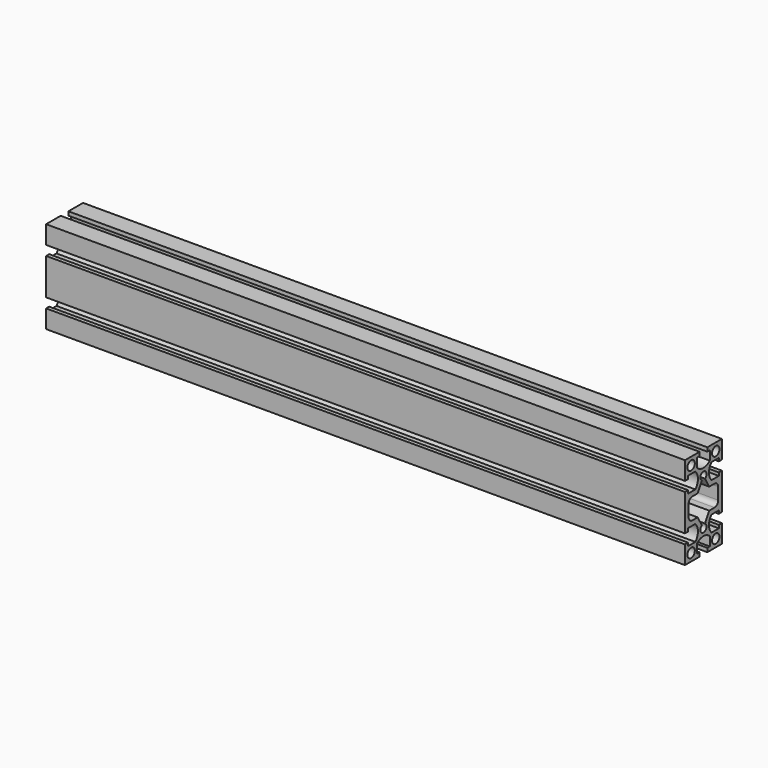
from build123d import *

# Parameters (mm, degrees)
F0_R     = 3
F1_DEPTH = 415


# Not quite as in the source:
# - ends of sketch curves that miss each other by under 0.0002 mm in the source are joined


with BuildPart() as f1:
    # F0 (on Right) → F1 (new body)
    with BuildSketch(Plane.YZ):
        with BuildLine():
            Line((12.5, -11.85), (15, -11.85))
            Line((15, -11.85), (15, 11.85))
            Line((15, 11.85), (12.5, 11.85))
            Line((12.5, 11.85), (12.5, 9.85))
            Line((12.5, 9.85), (6.547707, 9.85))
            ThreePointArc((6.5477069495, 9.8499999523), (4.5, 15), (6.5477069495, 20.1500000477))
            Line((6.547707, 20.15), (12.5, 20.15))
            Line((12.5, 20.15), (12.5, 18.15))
            Line((12.5, 18.15), (15, 18.15))
            Line((15, 18.15), (15, 30))
            Line((15, 30), (3.15, 30))
            Line((3.15, 30), (3.15, 27.5))
            Line((3.15, 27.5), (5.15, 27.5))
            Line((5.15, 27.5), (5.15, 21.547707))
            ThreePointArc((5.1500000477, 21.5477069495), (0, 19.5), (-5.1500000477, 21.5477069495))
            Line((-5.15, 21.547707), (-5.15, 27.5))
            Line((-5.15, 27.5), (-3.15, 27.5))
            Line((-3.15, 27.5), (-3.15, 30))
            Line((-3.15, 30), (-15, 30))
            Line((-15, 30), (-15, 18.15))
            Line((-15, 18.15), (-12.5, 18.15))
            Line((-12.5, 18.15), (-12.5, 20.15))
            Line((-12.5, 20.15), (-6.547707, 20.15))
            ThreePointArc((-6.5477069495, 20.1500000477), (-4.5, 15), (-6.5477069495, 9.8499999523))
            Line((-6.547707, 9.85), (-12.5, 9.85))
            Line((-12.5, 9.85), (-12.5, 11.85))
            Line((-12.5, 11.85), (-15, 11.85))
            Line((-15, 11.85), (-15, -11.85))
            Line((-15, -11.85), (-12.5, -11.85))
            Line((-12.5, -11.85), (-12.5, -9.85))
            Line((-12.5, -9.85), (-6.547707, -9.85))
            ThreePointArc((-6.5477069495, -9.8499999523), (-4.5, -15), (-6.5477069495, -20.1500000477))
            Line((-6.547707, -20.15), (-12.5, -20.15))
            Line((-12.5, -20.15), (-12.5, -18.15))
            Line((-12.5, -18.15), (-15, -18.15))
            Line((-15, -18.15), (-15, -30))
            Line((-15, -30), (-3.15, -30))
            Line((-3.15, -30), (-3.15, -27.5))
            Line((-3.15, -27.5), (-5.15, -27.5))
            Line((-5.15, -27.5), (-5.15, -21.547707))
            ThreePointArc((-5.1500000477, -21.5477069495), (0, -19.5), (5.1500000477, -21.5477069495))
            Line((5.15, -21.547707), (5.15, -27.5))
            Line((5.15, -27.5), (3.15, -27.5))
            Line((3.15, -27.5), (3.15, -30))
            Line((3.15, -30), (15, -30))
            Line((15, -30), (15, -18.15))
            Line((15, -18.15), (12.5, -18.15))
            Line((12.5, -18.15), (12.5, -20.15))
            Line((12.5, -20.15), (6.547707, -20.15))
            ThreePointArc((6.5477069495, -20.1500000477), (4.5, -15), (6.5477069495, -9.8499999523))
            Line((6.547707, -9.85), (12.5, -9.85))
            Line((12.5, -9.85), (12.5, -11.85))
        make_face()
        with Locations((-10, -25)):
            Circle(F0_R, mode=Mode.SUBTRACT)
        with Locations((10, -25)):
            Circle(F0_R, mode=Mode.SUBTRACT)
        with Locations((-10, 25)):
            Circle(F0_R, mode=Mode.SUBTRACT)
        with BuildLine():
            ThreePointArc((-12, 3.85), (-11.1213203436, 5.9713203436), (-9, 6.85))
            Line((-9, 6.85), (-4.705405, 6.85))
            Line((-4.705405, 6.85), (-1.25, 12.834936))
            ThreePointArc((-1.25, 12.834936), (0, 17.5), (1.2499997876, 12.8349363679))
            Line((1.2499997876, 12.8349363679), (4.705405, 6.85))
            Line((4.705405, 6.85), (9, 6.85))
            ThreePointArc((9, 6.85), (11.1213203436, 5.9713203436), (12, 3.85))
            Line((12, 3.85), (12, -3.85))
            ThreePointArc((12, -3.85), (11.1213203436, -5.9713203436), (9, -6.85))
            Line((9, -6.85), (4.705405, -6.85))
            Line((4.705405, -6.85), (1.25, -12.834937))
            ThreePointArc((1.25, -12.834937), (0, -17.5), (-1.2500002206, -12.8349366179))
            Line((-1.2500002206, -12.8349366179), (-4.705405, -6.85))
            Line((-4.705405, -6.85), (-9, -6.85))
            ThreePointArc((-9, -6.85), (-11.1213203436, -5.9713203436), (-12, -3.85))
            Line((-12, -3.85), (-12, 3.85))
        make_face(mode=Mode.SUBTRACT)
        with Locations((10, 25)):
            Circle(F0_R, mode=Mode.SUBTRACT)
    extrude(amount=F1_DEPTH)


solid = f1.part
